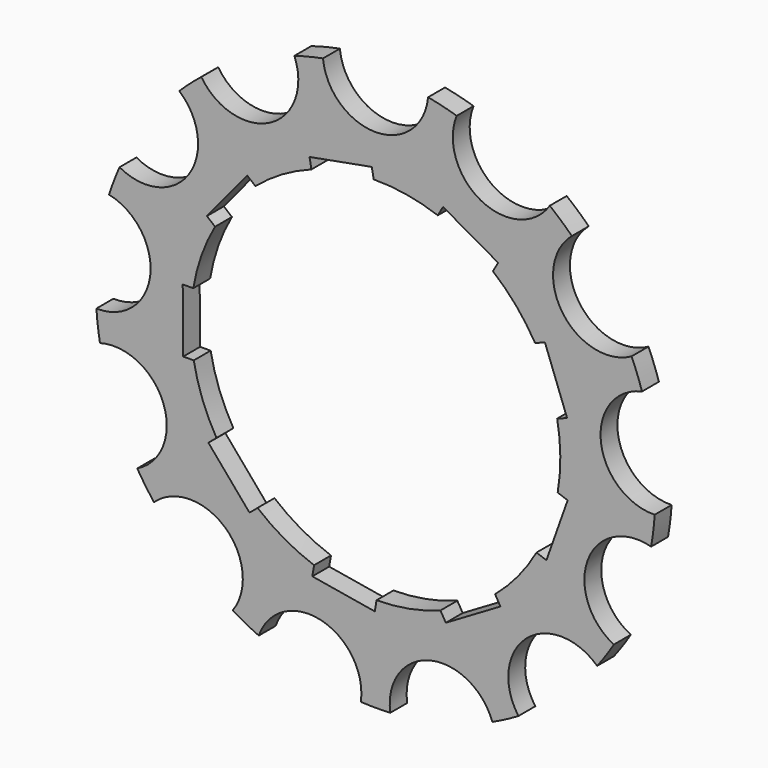
from build123d import *

# Parameters (mm, degrees)
F0_R            = 26.5
F0_R_2          = 17.5
F1_DEPTH        = 2
F3_DEPTH        = 2.001
F3_COPIES_COUNT = 13
F6_DEPTH        = 25
F6_COPIES_COUNT = 9


# Not quite as in the source:
# - a pattern or mirror of a feature is missing from the dataset's text; its kind, count and spacing are read off the source's solid


with BuildPart() as f1:
    # F0 (on Front) → F1 (new body)
    with BuildSketch(Plane.XZ):
        Circle(F0_R)
        Circle(F0_R_2, mode=Mode.SUBTRACT)
    extrude(amount=F1_DEPTH)

    # F2 (on face) → F3 (cut, through all)
    with BuildSketch(Plane.XZ.offset(2)):
        with BuildLine():
            ThreePointArc((4.9777003616, 26.0283018868), (0, 26.5), (-4.9777003616, 26.0283018868))
            ThreePointArc((-4.9777003616, 26.0283018868), (0, 21.5), (4.9777003616, 26.0283018868))
        make_face()
    f3 = extrude(amount=-F3_DEPTH, mode=Mode.SUBTRACT)

    # F3_copies: F3 ×13 about axis
    f3_copies_axis = Axis((0, 0, 0), (0, 1, 0))
    for i in range(1, F3_COPIES_COUNT):
        add(f3.rotate(f3_copies_axis, i * 360 / F3_COPIES_COUNT), mode=Mode.SUBTRACT)

    # F5 (on face) → F6 (cut)
    with BuildSketch(Plane.XZ.offset(2)):
        with BuildLine():
            Line((-6.2547624065, 17.3956841353), (-6.0736095937, 16.4122291753))
            ThreePointArc((-6.0736095937, 16.4122291753), (-3.1701742248, 17.2104618004), (-0.1728798335, 17.4991460524))
            Line((-0.1728798335, 17.4991460524), (-0.3540326464, 18.4826010124))
            Line((-0.3540326464, 18.4826010124), (-6.2547624065, 17.3956841353))
        make_face()
    f6 = extrude(amount=-F6_DEPTH, mode=Mode.SUBTRACT)

    # F6_copies: F6 ×9 about axis
    f6_copies_axis = Axis((0, 0, 0), (0, 1, 0))
    for i in range(1, F6_COPIES_COUNT):
        add(f6.rotate(f6_copies_axis, i * 360 / F6_COPIES_COUNT), mode=Mode.SUBTRACT)


solid = f1.part
